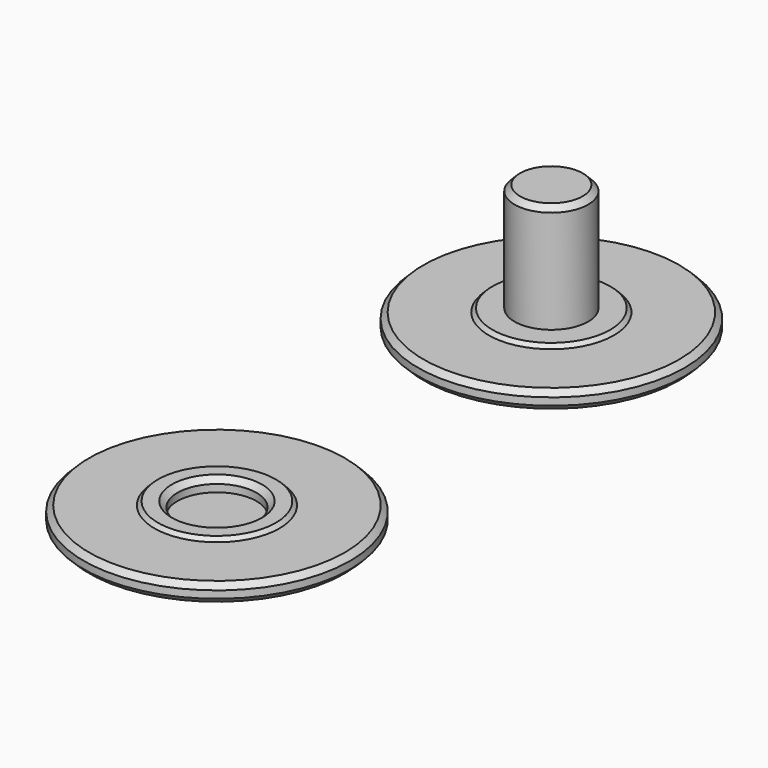
from build123d import *

# Parameters (mm, degrees)
F0_R     = 7.25
F0_R_2   = 3.1
F1_DEPTH = 1
F0_R_3   = 2
F2_DEPTH = 1.2
F0_R_4   = 2.15
F3_DEPTH = 7.1
F4_DEPTH = 0.5


# Not quite as in the source:
# - a fillet or chamfer that OpenCascade refuses, or shapes differently, is made with other operations: its cross-section is extruded or revolved along the edge and cut away or added


with BuildPart() as f1:
    # F0 (on Top) → F1 (new body)
    with BuildSketch(Plane.XY):
        Circle(F0_R)
        Circle(F0_R_2, mode=Mode.SUBTRACT)
    extrude(amount=F1_DEPTH)

    # F0 (on Top) → F2 (join)
    with BuildSketch(Plane.XY):
        Circle(F0_R_2)
        Circle(F0_R_3, mode=Mode.SUBTRACT)
    extrude(amount=F2_DEPTH)

    # F0 (on Top) → F3 (join)
    with BuildSketch(Plane.XY):
        Circle(F0_R_3)
    extrude(amount=F3_DEPTH)

    # F5#2: chamfer of 0.3 on 4 edges, made by hand


with BuildPart() as f1b:
    # F0 (on Top) → F1, piece 2 (new body)
    with BuildSketch(Plane.XY):
        with Locations((0, -22.7162558585)):
            Circle(F0_R)
        with Locations((0, -22.7162558585)):
            Circle(F0_R_2, mode=Mode.SUBTRACT)
    extrude(amount=F1_DEPTH)

    # F0 (on Top) → F2, piece 2 (join)
    with BuildSketch(Plane.XY):
        with Locations((0, -22.7162558585)):
            Circle(F0_R_2)
        with Locations((0, -22.7162558585)):
            Circle(F0_R_4, mode=Mode.SUBTRACT)
    extrude(amount=F2_DEPTH)

    # F0 (on Top) → F4 (join)
    with BuildSketch(Plane.XY):
        with Locations((0, -22.7162558585)):
            Circle(F0_R_4)
    extrude(amount=F4_DEPTH)

    # F5: chamfer of 0.3 on 4 edges, made by hand


with BuildPart() as f5_tool2:
    # F5_s3 → F5_t4 (revolve)
    with BuildSketch(Plane.XZ.offset(22.7162558585)):
        Polygon((3.4, 1), (3.1, 1.3), (3.1, 1), align=None)
    revolve(axis=Axis((0, -22.7162558585, 1), (0, 0, 1)))

    split(bisect_by=Plane.XY.offset(1.2), keep=Keep.BOTTOM)


with BuildPart() as f1b_1:
    add(f1b.part)

    # F5_t1: union F5_tool2
    add(f5_tool2.part)

    # F5_s6 → F5_t7 (revolve, cut)
    with BuildSketch(Plane.XZ.offset(22.7162558585)):
        Polygon((7.25, 0.3), (6.95, 0), (7.25, 0), align=None)
    revolve(axis=Axis((0, -22.7162558585, 0), (0, 0, 1)), mode=Mode.SUBTRACT)

    # F5_s8 → F5_t9 (revolve, cut)
    with BuildSketch(Plane.XZ.offset(22.7162558585)):
        Polygon((7.25, 0.7), (6.95, 1), (7.25, 1), align=None)
    revolve(axis=Axis((0, -22.7162558585, 1), (0, 0, 1)), mode=Mode.SUBTRACT)

    # F5_s10 → F5_t11 (revolve, cut)
    with BuildSketch(Plane.XZ.offset(22.7162558585)):
        Polygon((2.45, 1.2), (2.15, 0.9), (2.15, 1.2), align=None)
    revolve(axis=Axis((0, -22.7162558585, 1.2), (0, 0, 1)), mode=Mode.SUBTRACT)


with BuildPart() as f5_2_tool2:
    # F5_2_s3 → F5_2_t4 (revolve)
    with BuildSketch(Plane.XZ):
        Polygon((3.4, 1), (3.1, 1.3), (3.1, 1), align=None)
    revolve(axis=Axis((0, 0, 1), (0, 0, 1)))

    split(bisect_by=Plane.XY.offset(1.2), keep=Keep.BOTTOM)


with BuildPart() as f1_1:
    add(f1.part)

    # F5_2_t1: union F5_2_tool2
    add(f5_2_tool2.part)

    # F5_2_s6 → F5_2_t7 (revolve, cut)
    with BuildSketch(Plane.XZ):
        Polygon((7.25, 0.3), (6.95, 0), (7.25, 0), align=None)
    revolve(axis=Axis((0, 0, 0), (0, 0, 1)), mode=Mode.SUBTRACT)

    # F5_2_s8 → F5_2_t9 (revolve, cut)
    with BuildSketch(Plane.XZ):
        Polygon((7.25, 0.7), (6.95, 1), (7.25, 1), align=None)
    revolve(axis=Axis((0, 0, 1), (0, 0, 1)), mode=Mode.SUBTRACT)

    # F5_2_s10 → F5_2_t11 (revolve, cut)
    with BuildSketch(Plane.XZ):
        Polygon((2, 6.8), (1.7, 7.1), (2, 7.1), align=None)
    revolve(axis=Axis((0, 0, 7.1), (0, 0, 1)), mode=Mode.SUBTRACT)


solid = Compound([f1b_1.part, f1_1.part])
